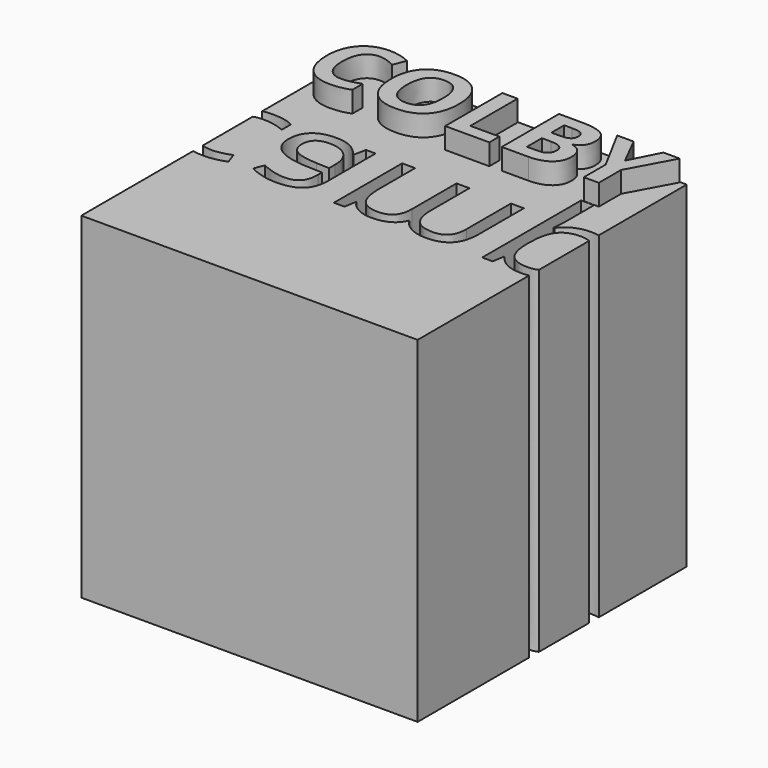
from build123d import *

# Parameters (mm, degrees)
F0_W         = 101.6
F0_H         = 101.6
F1_DEPTH     = 50.8
F2_TEXT_SIZE = 30.2479415732
F3_DEPTH     = 6.35
F4_TEXT_SIZE = 48.157091799
F5_DEPTH     = 121.666


# Not quite as in the source:
# - Text() gives the source's letters only with a copy of the font that has no kerning and outlines rounded to 1/6400 em; it was checked with that copy


with BuildPart() as f1:
    # F0 (on Front) → F1 (new body, symmetric)
    with BuildSketch(Plane.XZ):
        Rectangle(F0_W, F0_H)
    extrude(amount=F1_DEPTH, both=True)

    # F2 (on face) → F3 (join)
    with BuildSketch(Plane.XY.offset(50.8)):
        with Locations((-50.8, 29.0214820673)):
            Text('COLBY', F2_TEXT_SIZE, font='Open Sans', font_style=FontStyle.BOLD, text_align=(TextAlign.LEFT, TextAlign.BOTTOM))
    extrude(amount=F3_DEPTH)

    # F4 (on face) → F5 (cut)
    with BuildSketch(Plane(origin=(0, 0, -50.8), x_dir=(1, 0, 0), z_dir=(0, 0, -1))):
        with Locations((-62.227992059, -17.3365530476)):
            Text('camp', F4_TEXT_SIZE, font='Open Sans', text_align=(TextAlign.LEFT, TextAlign.BOTTOM))
    extrude(amount=-F5_DEPTH, mode=Mode.SUBTRACT)


solid = f1.part
